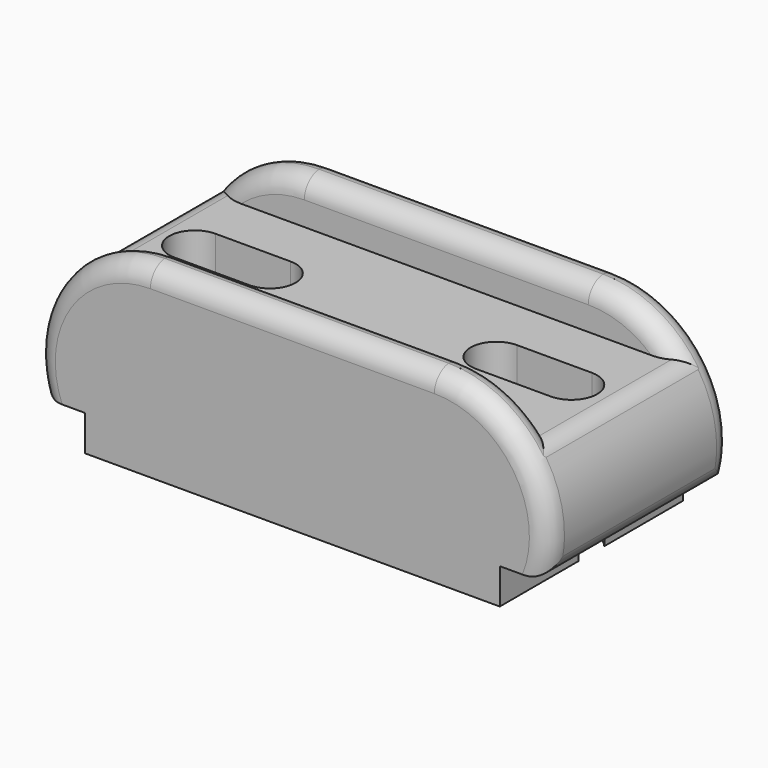
from build123d import *

# Parameters (mm, degrees)
F1_DEPTH      = 29
F2_W          = 39.6956643381
F2_H          = 11
F3_DEPTH      = 64.9329024958
F3_DEPTH_BACK = 94
F5_DEPTH      = 36.001
F6_T1_DEPTH   = 71.8638049916
F6_T3_DEPTH   = 39.6956643381
F6_T5_DEPTH   = 79.4647888213
F6_T10_ANGLE  = 76.3379776267
F6_T15_ANGLE  = 76.3379776267
F6_T18_ANGLE  = 132.7955508157
F6_T20_ANGLE  = 132.7955508157
F6_T22_ANGLE  = 132.7955508157
F6_T26_ANGLE  = 76.3379776267
F6_T31_ANGLE  = 76.3379776267
F6_T34_ANGLE  = 132.7955508157
F6_T39_ANGLE  = 76.3379776267
F6_T43_DEPTH  = 46.7434777317
F6_T50_DEPTH  = 46.7434777317
F6_T54_ANGLE  = 76.3379776267
F6_T61_ANGLE  = 76.3379776267
F6_T65_DEPTH  = 46.7434777317
F6_T72_DEPTH  = 46.7434777317
F6_T76_ANGLE  = 76.3379776267


# Not quite as in the source:
# - a fillet or chamfer that OpenCascade refuses, or shapes differently, is made with other operations: its cross-section is extruded or revolved along the edge and cut away or added


with BuildPart() as f1:
    # F0 (on Front) → F1 (new body, symmetric)
    with BuildSketch(Plane.XZ):
        with BuildLine():
            Line((-52.5, 9), (-52.5, 0))
            Line((-52.5, 0), (52.5, 0))
            Line((52.5, 0), (52.5, 9))
            Line((52.5, 9), (63.5, 9))
            ThreePointArc((63.5, 9), (59.4052916844, 35.0293863659), (35.9319024958, 47))
            Line((35.9319024958, 47), (-35.9319024958, 47))
            ThreePointArc((-35.9319024958, 47), (-59.4052916844, 35.0293863659), (-63.5, 9))
            Line((-63.5, 9), (-52.5, 9))
        make_face()
    extrude(amount=F1_DEPTH, both=True)

    # F2 (on Right) → F3 (cut, two sides)
    with BuildSketch(Plane.YZ) as f3_sk:
        with Locations((-0.1597600058, 41.5)):
            Rectangle(F2_W, F2_H)
    extrude(amount=-F3_DEPTH, mode=Mode.SUBTRACT)
    extrude(f3_sk.sketch, amount=F3_DEPTH_BACK, mode=Mode.SUBTRACT)

    # F4 (on face) → F5 (cut, through all)
    with BuildSketch(Plane.XY.offset(36)):
        with BuildLine():
            Line((-47.8754565308, -6.5), (-28.8754565308, -6.5))
            ThreePointArc((-28.8754565308, -6.5), (-22.3754565308, 0), (-28.8754565308, 6.5))
            Line((-28.8754565308, 6.5), (-47.8754565308, 6.5))
            ThreePointArc((-47.8754565308, 6.5), (-54.3754565308, 0), (-47.8754565308, -6.5))
        make_face()
        with BuildLine():
            Line((28.4296313102, -6.5), (47.4296313102, -6.5))
            ThreePointArc((47.4296313102, -6.5), (53.9296313102, 0), (47.4296313102, 6.5))
            Line((47.4296313102, 6.5), (28.4296313102, 6.5))
            ThreePointArc((28.4296313102, 6.5), (21.9296313102, 0), (28.4296313102, -6.5))
        make_face()
    extrude(amount=-F5_DEPTH, mode=Mode.SUBTRACT)

    # F6: fillet of radius 5 on 18 edges, made by hand

    # F6_s2 → F6_t1 (cut)
    with BuildSketch(Plane.YZ.offset(-35.9319024958)):
        with BuildLine():
            ThreePointArc((24.6890378487, 47.0004), (21.1525382574, 45.5355339059), (19.6876721633, 41.9990343146))
            Line((19.6876721633, 41.9990343146), (19.1875355947, 41.9990343146))
            ThreePointArc((19.1875355947, 41.9990343146), (19.1879355947, 44.4995171573), (19.1879355947, 47))
            Line((19.1879355947, 47), (19.6880721633, 47.5001365685))
            ThreePointArc((19.6880721633, 47.5001365685), (22.188555006, 47.5001365685), (24.6890378487, 47.5005365685))
            Line((24.6890378487, 47.5005365685), (24.6890378487, 47.0004))
        make_face()
        with BuildLine():
            ThreePointArc((23.9990343146, 47.0004), (27.5355339059, 45.5355339059), (29.0004, 41.9990343146))
            Line((29.0004, 41.9990343146), (29.5005365685, 41.9990343146))
            ThreePointArc((29.5005365685, 41.9990343146), (29.5001365685, 44.4995171573), (29.5001365685, 47))
            Line((29.5001365685, 47), (29, 47.5001365685))
            ThreePointArc((29, 47.5001365685), (26.4995171573, 47.5001365685), (23.9990343146, 47.5005365685))
            Line((23.9990343146, 47.5005365685), (23.9990343146, 47.0004))
        make_face()
        with BuildLine():
            ThreePointArc((-25.0085578603, 47.0004), (-21.4720582689, 45.5355339059), (-20.0071921748, 41.9990343146))
            Line((-20.0071921748, 41.9990343146), (-19.5070556063, 41.9990343146))
            ThreePointArc((-19.5070556063, 41.9990343146), (-19.5074556063, 44.4995171573), (-19.5074556063, 47))
            Line((-19.5074556063, 47), (-20.0075921748, 47.5001365685))
            ThreePointArc((-20.0075921748, 47.5001365685), (-22.5080750175, 47.5001365685), (-25.0085578603, 47.5005365685))
            Line((-25.0085578603, 47.5005365685), (-25.0085578603, 47.0004))
        make_face()
        with BuildLine():
            ThreePointArc((-29.0004, 41.9990343146), (-27.5355339059, 45.5355339059), (-23.9990343146, 47.0004))
            Line((-23.9990343146, 47.0004), (-23.9990343146, 47.5005365685))
            ThreePointArc((-23.9990343146, 47.5005365685), (-26.4995171573, 47.5001365685), (-29, 47.5001365685))
            Line((-29, 47.5001365685), (-29.5001365685, 47))
            ThreePointArc((-29.5001365685, 47), (-29.5001365685, 44.4995171573), (-29.5005365685, 41.9990343146))
            Line((-29.5005365685, 41.9990343146), (-29.0004, 41.9990343146))
        make_face()
    extrude(amount=F6_T1_DEPTH, mode=Mode.SUBTRACT)

    # F6_s4 → F6_t3 (cut)
    with BuildSketch(Plane.XZ.offset(-19.6880721633)):
        with BuildLine():
            ThreePointArc((-60.3101603912, 33.7074422535), (-58.4998694367, 35.3899084513), (-56.1050529687, 36.0004))
            Line((-56.1050529687, 36.0004), (-56.1050529687, 36.50064))
            ThreePointArc((-56.1050529687, 36.50064), (-57.3872947331, 36.50024), (-58.6695364976, 36.50024))
            Line((-58.6695364976, 36.50024), (-59.0617528436, 36.3104937931))
            ThreePointArc((-59.0617528436, 36.3104937931), (-59.9244071951, 35.1646112194), (-60.7306711334, 33.9783864789))
            Line((-60.7306711334, 33.9783864789), (-60.3101603912, 33.7074422535))
        make_face()
        with BuildLine():
            ThreePointArc((60.3101603912, 33.7074422535), (58.4998694367, 35.3899084513), (56.1050529687, 36.0004))
            Line((56.1050529687, 36.0004), (56.1050529687, 36.50064))
            ThreePointArc((56.1050529687, 36.50064), (57.3872947331, 36.50024), (58.6695364976, 36.50024))
            Line((58.6695364976, 36.50024), (59.0617528436, 36.3104937931))
            ThreePointArc((59.0617528436, 36.3104937931), (59.9244071951, 35.1646112194), (60.7306711334, 33.9783864789))
            Line((60.7306711334, 33.9783864789), (60.3101603912, 33.7074422535))
        make_face()
    extrude(amount=F6_T3_DEPTH, mode=Mode.SUBTRACT)

    # F6_s6 → F6_t5 (cut)
    with BuildSketch(Plane.XZ.offset(-39.7323944107)):
        with BuildLine():
            ThreePointArc((-64.526971658, 13.1683108784), (-62.8237409902, 10.1813793629), (-59.594785722, 8.9996))
            Line((-59.594785722, 8.9996), (-59.594785722, 8.4993901064))
            ThreePointArc((-59.594785722, 8.4993901064), (-61.547392861, 8.4997901064), (-63.5, 8.4997901064))
            Line((-63.5, 8.4997901064), (-63.9755115558, 8.8447624468))
            ThreePointArc((-63.9755115558, 8.8447624468), (-64.576227141, 10.945565268), (-65.0201902516, 13.0849720727))
            Line((-65.0201902516, 13.0849720727), (-64.526971658, 13.1683108784))
        make_face()
        with BuildLine():
            ThreePointArc((64.526971658, 13.1683108784), (62.8237409902, 10.1813793629), (59.594785722, 8.9996))
            Line((59.594785722, 8.9996), (59.594785722, 8.4993901064))
            ThreePointArc((59.594785722, 8.4993901064), (61.547392861, 8.4997901064), (63.5, 8.4997901064))
            Line((63.5, 8.4997901064), (63.9755115558, 8.8447624468))
            ThreePointArc((63.9755115558, 8.8447624468), (64.576227141, 10.945565268), (65.0201902516, 13.0849720727))
            Line((65.0201902516, 13.0849720727), (64.526971658, 13.1683108784))
        make_face()
    extrude(amount=F6_T5_DEPTH, mode=Mode.SUBTRACT)


with BuildPart() as f6_tool8:
    # F6_s9 → F6_t10 (revolve)
    with BuildSketch(Plane.YZ.offset(-35.9319024958)):
        with BuildLine():
            ThreePointArc((19.6876721633, 41.9990343146), (21.1525382574, 45.5355339059), (24.6890378487, 47.0004))
            Line((24.6890378487, 47.0004), (24.6890378487, 47.5005365685))
            ThreePointArc((24.6890378487, 47.5005365685), (22.188555006, 47.5001365685), (19.6880721633, 47.5001365685))
            Line((19.6880721633, 47.5001365685), (19.1879355947, 47))
            ThreePointArc((19.1879355947, 47), (19.1879355947, 44.4995171573), (19.1875355947, 41.9990343146))
            Line((19.1875355947, 41.9990343146), (19.6876721633, 41.9990343146))
        make_face()
    revolve(axis=Axis((-35.9319024958, 19.6880721633, 18), (0, -1, 0)), revolution_arc=F6_T10_ANGLE)

    split(bisect_by=Plane.XY.offset(36), keep=Keep.TOP)


with BuildPart() as f1_1:
    add(f1.part)

    # F6_t7: cut F6_tool8
    add(f6_tool8.part, mode=Mode.SUBTRACT)


with BuildPart() as f6_tool13:
    # F6_s14 → F6_t15 (revolve)
    with BuildSketch(Plane.YZ.offset(-35.9319024958)):
        with BuildLine():
            ThreePointArc((-25.0085578603, 47.0004), (-21.4720582689, 45.5355339059), (-20.0071921748, 41.9990343146))
            Line((-20.0071921748, 41.9990343146), (-19.5070556063, 41.9990343146))
            ThreePointArc((-19.5070556063, 41.9990343146), (-19.5074556063, 44.4995171573), (-19.5074556063, 47))
            Line((-19.5074556063, 47), (-20.0075921748, 47.5001365685))
            ThreePointArc((-20.0075921748, 47.5001365685), (-22.5080750175, 47.5001365685), (-25.0085578603, 47.5005365685))
            Line((-25.0085578603, 47.5005365685), (-25.0085578603, 47.0004))
        make_face()
    revolve(axis=Axis((-35.9319024958, -20.0075921748, 18), (0, -1, 0)), revolution_arc=F6_T15_ANGLE)

    split(bisect_by=Plane.XY.offset(36), keep=Keep.TOP)


with BuildPart() as f1_2:
    add(f1_1.part)

    # F6_t12: cut F6_tool13
    add(f6_tool13.part, mode=Mode.SUBTRACT)

    # F6_s17 → F6_t18 (revolve, cut)
    with BuildSketch(Plane.YZ.offset(-35.9319024958)):
        with BuildLine():
            ThreePointArc((-23.9990343146, 47.0004), (-27.5355339059, 45.5355339059), (-29.0004, 41.9990343146))
            Line((-29.0004, 41.9990343146), (-29.5005365685, 41.9990343146))
            ThreePointArc((-29.5005365685, 41.9990343146), (-29.5001365685, 44.4995171573), (-29.5001365685, 47))
            Line((-29.5001365685, 47), (-29, 47.5001365685))
            ThreePointArc((-29, 47.5001365685), (-26.4995171573, 47.5001365685), (-23.9990343146, 47.5005365685))
            Line((-23.9990343146, 47.5005365685), (-23.9990343146, 47.0004))
        make_face()
    revolve(axis=Axis((-35.9319024958, -29, 18), (0, -1, 0)), revolution_arc=F6_T18_ANGLE, mode=Mode.SUBTRACT)

    # F6_s19 → F6_t20 (revolve, cut)
    with BuildSketch(Plane.YZ.offset(-35.9319024958)):
        with BuildLine():
            ThreePointArc((23.9990343146, 47.0004), (27.5355339059, 45.5355339059), (29.0004, 41.9990343146))
            Line((29.0004, 41.9990343146), (29.5005365685, 41.9990343146))
            ThreePointArc((29.5005365685, 41.9990343146), (29.5001365685, 44.4995171573), (29.5001365685, 47))
            Line((29.5001365685, 47), (29, 47.5001365685))
            ThreePointArc((29, 47.5001365685), (26.4995171573, 47.5001365685), (23.9990343146, 47.5005365685))
            Line((23.9990343146, 47.5005365685), (23.9990343146, 47.0004))
        make_face()
    revolve(axis=Axis((-35.9319024958, 29, 18), (0, -1, 0)), revolution_arc=F6_T20_ANGLE, mode=Mode.SUBTRACT)

    # F6_s21 → F6_t22 (revolve, cut)
    with BuildSketch(Plane(origin=(25.5582063795, 0, 27.6046517371), x_dir=(0, 1, 0), z_dir=(-0.679384326, 0, -0.7337826229))):
        with BuildLine():
            ThreePointArc((-23.9990343146, 43.1376877916), (-27.5355339059, 41.6728216976), (-29.0004, 38.1363221062))
            Line((-29.0004, 38.1363221062), (-29.5005365685, 38.1363221062))
            ThreePointArc((-29.5005365685, 38.1363221062), (-29.5001365685, 40.6368049489), (-29.5001365685, 43.1372877916))
            Line((-29.5001365685, 43.1372877916), (-29, 43.6374243602))
            ThreePointArc((-29, 43.6374243602), (-26.4995171573, 43.6374243602), (-23.9990343146, 43.6378243602))
            Line((-23.9990343146, 43.6378243602), (-23.9990343146, 43.1376877916))
        make_face()
    revolve(axis=Axis((35.9319024958, -29, 18), (0, -1, 0)), revolution_arc=F6_T22_ANGLE, mode=Mode.SUBTRACT)


with BuildPart() as f6_tool24:
    # F6_s25 → F6_t26 (revolve)
    with BuildSketch(Plane(origin=(-2.1266450769, 0, 8.7490474774), x_dir=(0, 1, 0), z_dir=(0.2361941177, 0, -0.9717058911))):
        with BuildLine():
            ThreePointArc((-25.0085578603, 68.1671354515), (-21.4720582689, 66.7022693574), (-20.0071921748, 63.165769766))
            Line((-20.0071921748, 63.165769766), (-19.5070556063, 63.165769766))
            ThreePointArc((-19.5070556063, 63.165769766), (-19.5074556063, 65.6662526087), (-19.5074556063, 68.1667354515))
            Line((-19.5074556063, 68.1667354515), (-20.0075921748, 68.66687202))
            ThreePointArc((-20.0075921748, 68.66687202), (-22.5080750175, 68.66687202), (-25.0085578603, 68.66727202))
            Line((-25.0085578603, 68.66727202), (-25.0085578603, 68.1671354515))
        make_face()
    revolve(axis=Axis((35.9319024958, -20.0075921748, 18), (0, -1, 0)), revolution_arc=F6_T26_ANGLE)

    split(bisect_by=Plane.XY.offset(36), keep=Keep.TOP)


with BuildPart() as f1_3:
    add(f1_2.part)

    # F6_t23: cut F6_tool24
    add(f6_tool24.part, mode=Mode.SUBTRACT)


with BuildPart() as f6_tool29:
    # F6_s30 → F6_t31 (revolve)
    with BuildSketch(Plane(origin=(-2.1266450769, 0, 8.7490474774), x_dir=(0, 1, 0), z_dir=(0.2361941177, 0, -0.9717058911))):
        with BuildLine():
            ThreePointArc((24.6890378487, 68.1671354515), (21.1525382574, 66.7022693574), (19.6876721633, 63.165769766))
            Line((19.6876721633, 63.165769766), (19.1875355947, 63.165769766))
            ThreePointArc((19.1875355947, 63.165769766), (19.1879355947, 65.6662526087), (19.1879355947, 68.1667354515))
            Line((19.1879355947, 68.1667354515), (19.6880721633, 68.66687202))
            ThreePointArc((19.6880721633, 68.66687202), (22.188555006, 68.66687202), (24.6890378487, 68.66727202))
            Line((24.6890378487, 68.66727202), (24.6890378487, 68.1671354515))
        make_face()
    revolve(axis=Axis((35.9319024958, 19.6880721633, 18), (0, -1, 0)), revolution_arc=F6_T31_ANGLE)

    split(bisect_by=Plane.XY.offset(36), keep=Keep.TOP)


with BuildPart() as f1_4:
    add(f1_3.part)

    # F6_t28: cut F6_tool29
    add(f6_tool29.part, mode=Mode.SUBTRACT)

    # F6_s33 → F6_t34 (revolve, cut)
    with BuildSketch(Plane(origin=(25.5582063795, 0, 27.6046517371), x_dir=(0, 1, 0), z_dir=(-0.679384326, 0, -0.7337826229))):
        with BuildLine():
            ThreePointArc((23.9990343146, 43.1376877916), (27.5355339059, 41.6728216976), (29.0004, 38.1363221062))
            Line((29.0004, 38.1363221062), (29.5005365685, 38.1363221062))
            ThreePointArc((29.5005365685, 38.1363221062), (29.5001365685, 40.6368049489), (29.5001365685, 43.1372877916))
            Line((29.5001365685, 43.1372877916), (29, 43.6374243602))
            ThreePointArc((29, 43.6374243602), (26.4995171573, 43.6374243602), (23.9990343146, 43.6378243602))
            Line((23.9990343146, 43.6378243602), (23.9990343146, 43.1376877916))
        make_face()
    revolve(axis=Axis((35.9319024958, 29, 18), (0, -1, 0)), revolution_arc=F6_T34_ANGLE, mode=Mode.SUBTRACT)


with BuildPart() as f6_tool37:
    # F6_s38 → F6_t39 (revolve)
    with BuildSketch(Plane.YZ.offset(-35.9319024958)):
        with BuildLine():
            ThreePointArc((19.6876721633, 41.9990343146), (21.1525382574, 45.5355339059), (24.6890378487, 47.0004))
            Line((24.6890378487, 47.0004), (24.6890378487, 47.5005365685))
            ThreePointArc((24.6890378487, 47.5005365685), (22.188555006, 47.5001365685), (19.6880721633, 47.5001365685))
            Line((19.6880721633, 47.5001365685), (19.1879355947, 47))
            ThreePointArc((19.1879355947, 47), (19.1879355947, 44.4995171573), (19.1875355947, 41.9990343146))
            Line((19.1875355947, 41.9990343146), (19.6876721633, 41.9990343146))
        make_face()
    revolve(axis=Axis((-35.9319024958, 19.6880721633, 18), (0, -1, 0)), revolution_arc=F6_T39_ANGLE)

    split(bisect_by=Plane.XY.offset(36), keep=Keep.BOTTOM)


with BuildPart() as f6_tool41:
    # F6_s42 → F6_t43 (new body)
    with BuildSketch(Plane.XZ.offset(-26.7358855569)):
        with BuildLine():
            ThreePointArc((-60.3101603912, 33.7074422535), (-58.4998694367, 35.3899084513), (-56.1050529687, 36.0004))
            Line((-56.1050529687, 36.0004), (-56.1050529687, 36.50064))
            ThreePointArc((-56.1050529687, 36.50064), (-57.3872947331, 36.50024), (-58.6695364976, 36.50024))
            Line((-58.6695364976, 36.50024), (-59.0617528436, 36.3104937931))
            ThreePointArc((-59.0617528436, 36.3104937931), (-59.9244071951, 35.1646112194), (-60.7306711334, 33.9783864789))
            Line((-60.7306711334, 33.9783864789), (-60.3101603912, 33.7074422535))
        make_face()
    extrude(amount=F6_T43_DEPTH)

    split(bisect_by=Plane.XZ.offset(-19.6880721633), keep=Keep.BOTTOM)


with BuildPart() as f6_tool37_1:
    add(f6_tool37.part)

    # F6_t45: intersect F6_tool41
    add(f6_tool41.part, mode=Mode.INTERSECT)


with BuildPart() as f1_5:
    add(f1_4.part)

    # F6_t35: cut F6_tool37
    add(f6_tool37_1.part, mode=Mode.SUBTRACT)


with BuildPart() as f6_tool48:
    # F6_s49 → F6_t50 (new body)
    with BuildSketch(Plane.XZ.offset(-19.6880721633)):
        with BuildLine():
            ThreePointArc((-60.3101603912, 33.7074422535), (-58.4998694367, 35.3899084513), (-56.1050529687, 36.0004))
            Line((-56.1050529687, 36.0004), (-56.1050529687, 36.50064))
            ThreePointArc((-56.1050529687, 36.50064), (-57.3872947331, 36.50024), (-58.6695364976, 36.50024))
            Line((-58.6695364976, 36.50024), (-59.0617528436, 36.3104937931))
            ThreePointArc((-59.0617528436, 36.3104937931), (-59.9244071951, 35.1646112194), (-60.7306711334, 33.9783864789))
            Line((-60.7306711334, 33.9783864789), (-60.3101603912, 33.7074422535))
        make_face()
    extrude(amount=F6_T50_DEPTH)

    split(bisect_by=Plane.XZ.offset(20.0075921748), keep=Keep.TOP)


with BuildPart() as f6_tool52:
    # F6_s53 → F6_t54 (revolve)
    with BuildSketch(Plane.YZ.offset(-35.9319024958)):
        with BuildLine():
            ThreePointArc((-25.0085578603, 47.0004), (-21.4720582689, 45.5355339059), (-20.0071921748, 41.9990343146))
            Line((-20.0071921748, 41.9990343146), (-19.5070556063, 41.9990343146))
            ThreePointArc((-19.5070556063, 41.9990343146), (-19.5074556063, 44.4995171573), (-19.5074556063, 47))
            Line((-19.5074556063, 47), (-20.0075921748, 47.5001365685))
            ThreePointArc((-20.0075921748, 47.5001365685), (-22.5080750175, 47.5001365685), (-25.0085578603, 47.5005365685))
            Line((-25.0085578603, 47.5005365685), (-25.0085578603, 47.0004))
        make_face()
    revolve(axis=Axis((-35.9319024958, -20.0075921748, 18), (0, -1, 0)), revolution_arc=F6_T54_ANGLE)

    split(bisect_by=Plane.XY.offset(36), keep=Keep.BOTTOM)


with BuildPart() as f6_tool48_1:
    add(f6_tool48.part)

    # F6_t56: intersect F6_tool52
    add(f6_tool52.part, mode=Mode.INTERSECT)


with BuildPart() as f1_6:
    add(f1_5.part)

    # F6_t46: cut F6_tool48
    add(f6_tool48_1.part, mode=Mode.SUBTRACT)


with BuildPart() as f6_tool59:
    # F6_s60 → F6_t61 (revolve)
    with BuildSketch(Plane(origin=(-2.1266450769, 0, 8.7490474774), x_dir=(0, 1, 0), z_dir=(0.2361941177, 0, -0.9717058911))):
        with BuildLine():
            ThreePointArc((-25.0085578603, 68.1671354515), (-21.4720582689, 66.7022693574), (-20.0071921748, 63.165769766))
            Line((-20.0071921748, 63.165769766), (-19.5070556063, 63.165769766))
            ThreePointArc((-19.5070556063, 63.165769766), (-19.5074556063, 65.6662526087), (-19.5074556063, 68.1667354515))
            Line((-19.5074556063, 68.1667354515), (-20.0075921748, 68.66687202))
            ThreePointArc((-20.0075921748, 68.66687202), (-22.5080750175, 68.66687202), (-25.0085578603, 68.66727202))
            Line((-25.0085578603, 68.66727202), (-25.0085578603, 68.1671354515))
        make_face()
    revolve(axis=Axis((35.9319024958, -20.0075921748, 18), (0, -1, 0)), revolution_arc=F6_T61_ANGLE)

    split(bisect_by=Plane.XY.offset(36), keep=Keep.BOTTOM)


with BuildPart() as f6_tool63:
    # F6_s64 → F6_t65 (new body)
    with BuildSketch(Plane.XZ.offset(-19.6880721633)):
        with BuildLine():
            ThreePointArc((60.3101603912, 33.7074422535), (58.4998694367, 35.3899084513), (56.1050529687, 36.0004))
            Line((56.1050529687, 36.0004), (56.1050529687, 36.50064))
            ThreePointArc((56.1050529687, 36.50064), (57.3872947331, 36.50024), (58.6695364976, 36.50024))
            Line((58.6695364976, 36.50024), (59.0617528436, 36.3104937931))
            ThreePointArc((59.0617528436, 36.3104937931), (59.9244071951, 35.1646112194), (60.7306711334, 33.9783864789))
            Line((60.7306711334, 33.9783864789), (60.3101603912, 33.7074422535))
        make_face()
    extrude(amount=F6_T65_DEPTH)

    split(bisect_by=Plane.XZ.offset(20.0075921748), keep=Keep.TOP)


with BuildPart() as f6_tool59_1:
    add(f6_tool59.part)

    # F6_t67: intersect F6_tool63
    add(f6_tool63.part, mode=Mode.INTERSECT)


with BuildPart() as f1_7:
    add(f1_6.part)

    # F6_t57: cut F6_tool59
    add(f6_tool59_1.part, mode=Mode.SUBTRACT)


with BuildPart() as f6_tool70:
    # F6_s71 → F6_t72 (new body)
    with BuildSketch(Plane.XZ.offset(-26.7358855569)):
        with BuildLine():
            ThreePointArc((60.3101603912, 33.7074422535), (58.4998694367, 35.3899084513), (56.1050529687, 36.0004))
            Line((56.1050529687, 36.0004), (56.1050529687, 36.50064))
            ThreePointArc((56.1050529687, 36.50064), (57.3872947331, 36.50024), (58.6695364976, 36.50024))
            Line((58.6695364976, 36.50024), (59.0617528436, 36.3104937931))
            ThreePointArc((59.0617528436, 36.3104937931), (59.9244071951, 35.1646112194), (60.7306711334, 33.9783864789))
            Line((60.7306711334, 33.9783864789), (60.3101603912, 33.7074422535))
        make_face()
    extrude(amount=F6_T72_DEPTH)

    split(bisect_by=Plane.XZ.offset(-19.6880721633), keep=Keep.BOTTOM)


with BuildPart() as f6_tool74:
    # F6_s75 → F6_t76 (revolve)
    with BuildSketch(Plane(origin=(-2.1266450769, 0, 8.7490474774), x_dir=(0, 1, 0), z_dir=(0.2361941177, 0, -0.9717058911))):
        with BuildLine():
            ThreePointArc((24.6890378487, 68.1671354515), (21.1525382574, 66.7022693574), (19.6876721633, 63.165769766))
            Line((19.6876721633, 63.165769766), (19.1875355947, 63.165769766))
            ThreePointArc((19.1875355947, 63.165769766), (19.1879355947, 65.6662526087), (19.1879355947, 68.1667354515))
            Line((19.1879355947, 68.1667354515), (19.6880721633, 68.66687202))
            ThreePointArc((19.6880721633, 68.66687202), (22.188555006, 68.66687202), (24.6890378487, 68.66727202))
            Line((24.6890378487, 68.66727202), (24.6890378487, 68.1671354515))
        make_face()
    revolve(axis=Axis((35.9319024958, 19.6880721633, 18), (0, -1, 0)), revolution_arc=F6_T76_ANGLE)

    split(bisect_by=Plane.XY.offset(36), keep=Keep.BOTTOM)


with BuildPart() as f6_tool70_1:
    add(f6_tool70.part)

    # F6_t78: intersect F6_tool74
    add(f6_tool74.part, mode=Mode.INTERSECT)


with BuildPart() as f1_8:
    add(f1_7.part)

    # F6_t68: cut F6_tool70
    add(f6_tool70_1.part, mode=Mode.SUBTRACT)


solid = f1_8.part
